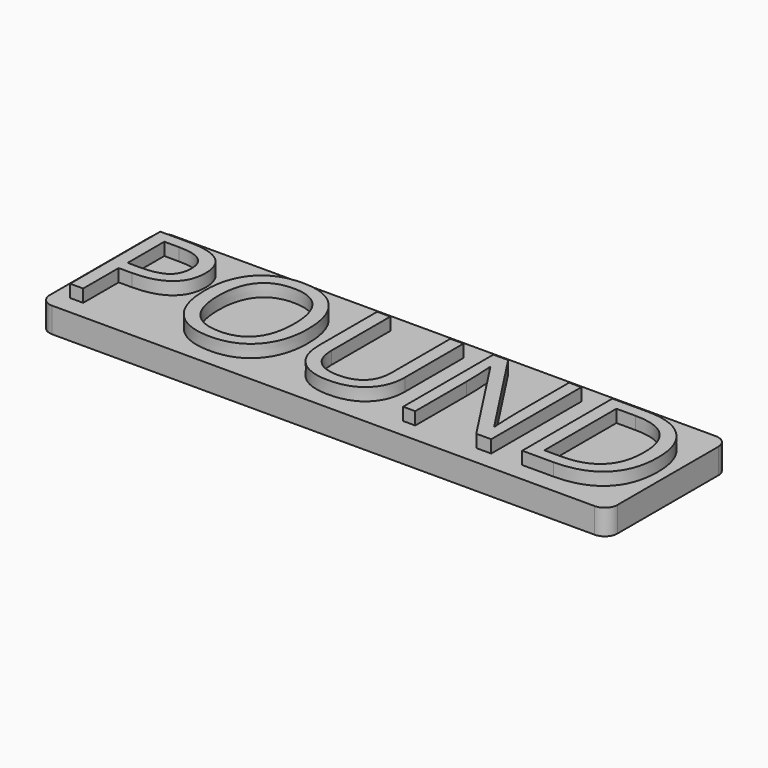
from build123d import *

# Parameters (mm, degrees)
F0_W         = 90
F0_H         = 24
F1_DEPTH     = 4
F2_R         = 2
F3_TEXT_SIZE = 25.0315066707
F4_DEPTH     = 2
F5_TEXT_SIZE = 17.3611111111
F6_DEPTH     = 1.5


# Not quite as in the source:
# - a feature names something its author has since deleted; it is built from what else it names
# - Text() gives the source's letters only with a copy of the font that has no kerning and outlines rounded to 1/6400 em; it was checked with that copy


with BuildPart() as f1:
    # F0 (on Top) → F1 (new body)
    with BuildSketch(Plane.XY):
        Rectangle(F0_W, F0_H)
    extrude(amount=F1_DEPTH)

    # F2
    f2_edges = [f1.edges().sort_by_distance(p)[0] for p in [
        (-45, -12, 2),
        (45, 12, 2),
        (-45, 12, 2),
        (45, -12, 2),
    ]]
    fillet(f2_edges, radius=F2_R)

    # F3 (on face) → F4 (join)
    with BuildSketch(Plane.XY.offset(4)):
        with Locations((-45, -9.0113424015)):
            Text('POUND', F3_TEXT_SIZE, font='Open Sans', text_align=(TextAlign.LEFT, TextAlign.BOTTOM))
    extrude(amount=F4_DEPTH)

    # F5 (on face) → F6 (cut)
    with BuildSketch(Plane(origin=(0, 0, 0), x_dir=(1, 0, 0), z_dir=(0, 0, -1))):
        with Locations((-34.0833875868, -6.25)):
            Text('0.454 kg', F5_TEXT_SIZE, font='Open Sans', text_align=(TextAlign.LEFT, TextAlign.BOTTOM))
    extrude(amount=-F6_DEPTH, mode=Mode.SUBTRACT)


solid = f1.part
